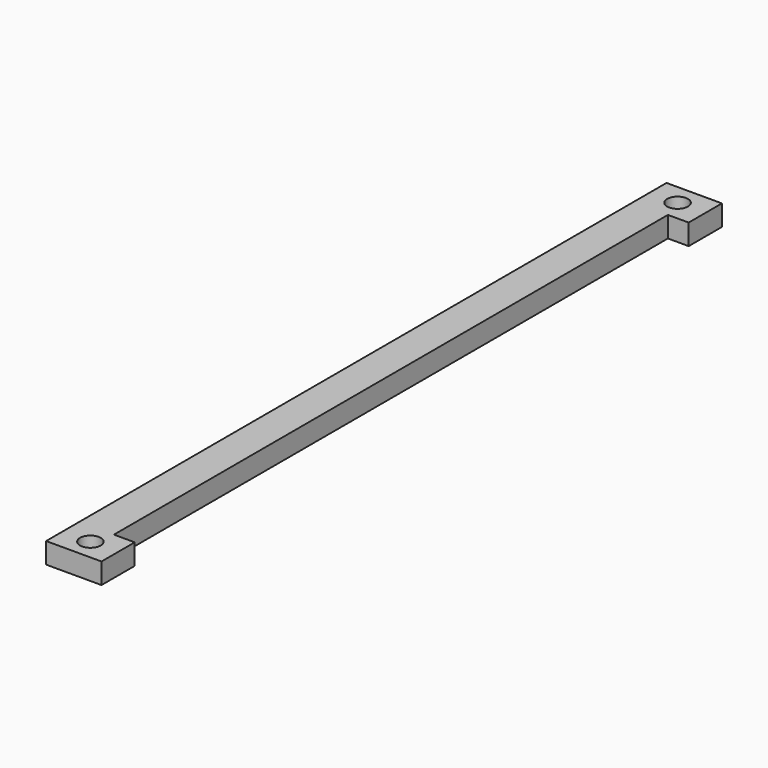
from build123d import *

# Parameters (mm, degrees)
F0_R     = 1.5
F1_DEPTH = 3


# Not quite as in the source:
# - a feature names something its author has since deleted; it is built from what else it names


with BuildPart() as f1:
    # F0 (on Top) → F1 (new body)
    with BuildSketch(Plane.XY):
        Polygon((-5, 59.4178017552), (-13, 59.4178017552), (-13, -52.5821982448), (-5, -52.5821982448), (-5, -46.5821982448), (-8, -46.5821982448), (-8, 53.4178017552), (-5, 53.4178017552), align=None)
        with Locations((-9, -49.5821982448)):
            Circle(F0_R, mode=Mode.SUBTRACT)
        with Locations((-9, 56.4178017552)):
            Circle(F0_R, mode=Mode.SUBTRACT)
    extrude(amount=F1_DEPTH)


solid = f1.part
